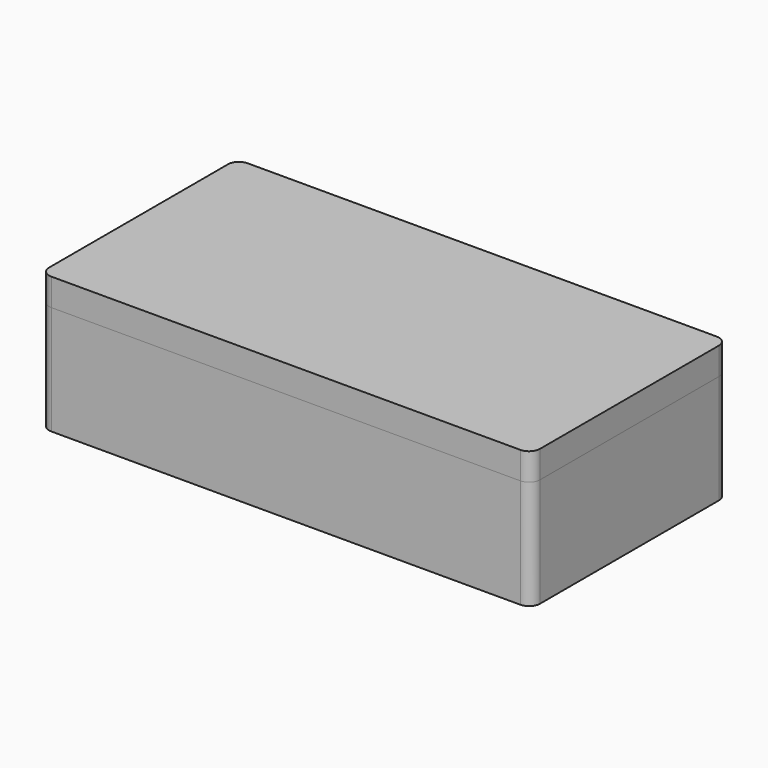
from build123d import *

# Parameters (mm, degrees)
F1_DEPTH = 500
F3_DEPTH = 400


# Not quite as in the source:
# - a feature names something its author has since deleted; it is built from what else it names


with BuildPart() as f1:
    # F0 (on Top) → F1 (new body)
    with BuildSketch(Plane.XY):
        with BuildLine():
            ThreePointArc((0, 40), (11.7157287525, 11.7157287525), (40, 0))
            Line((40, 0), (1760, 0))
            ThreePointArc((1760, 0), (1788.2842712475, 11.7157287525), (1800, 40))
            Line((1800, 40), (1800, 860))
            ThreePointArc((1800, 860), (1788.2842712475, 888.2842712475), (1760, 900))
            Line((1760, 900), (40, 900))
            ThreePointArc((40, 900), (11.7157287525, 888.2842712475), (0, 860))
            Line((0, 860), (0, 40))
        make_face()
    extrude(amount=F1_DEPTH)


with BuildPart() as f3:
    # F2 (on Top) → F3 (new body)
    with BuildSketch(Plane.XY):
        with BuildLine():
            ThreePointArc((40, 900), (11.7157287525, 888.2842712475), (0, 860))
            Line((0, 860), (0, 40))
            ThreePointArc((0, 40), (11.7157287525, 11.7157287525), (40, 0))
            Line((40, 0), (1760, 0))
            ThreePointArc((1760, 0), (1788.2842712475, 11.7157287525), (1800, 40))
            Line((1800, 40), (1800, 860))
            ThreePointArc((1800, 860), (1788.2842712475, 888.2842712475), (1760, 900))
            Line((1760, 900), (1660, 900))
            ThreePointArc((1660, 900), (1631.7157287525, 888.2842712475), (1620, 860))
            Line((1620, 860), (1620, 180))
            Line((1620, 180), (180, 180))
            Line((180, 180), (180, 860))
            ThreePointArc((180, 860), (168.2842712475, 888.2842712475), (140, 900))
            Line((140, 900), (40, 900))
        make_face()
    extrude(amount=F3_DEPTH)


solid = Compound([f1.part, f3.part])
